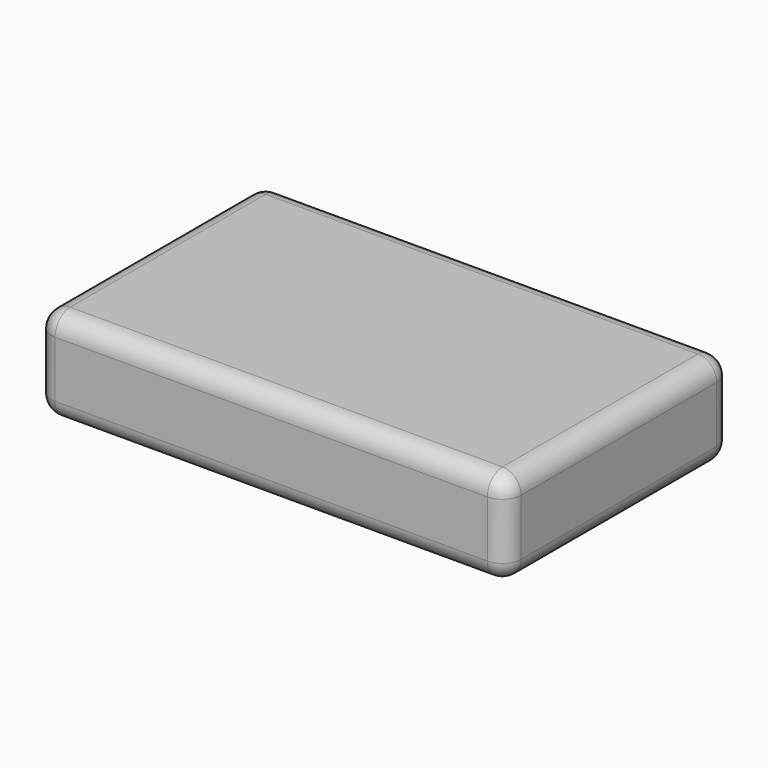
from build123d import *

# Parameters (mm, degrees)
F0_W         = 127
F0_H         = 76.2
F1_DEPTH     = 25.4
F2_R         = 5.08
F3_DEPTH     = 12.7
F4_W         = 101.6
F4_H         = 50.8
F5_DEPTH     = 12.7
F6_TEXT_SIZE = 70.5555555556
F7_DEPTH     = 22.86


# Not quite as in the source:
# - Text() gives the source's letters only with a copy of the font that has no kerning and outlines rounded to 1/6400 em; it was checked with that copy


with BuildPart() as f1:
    # F0 (on Top) → F1 (new body)
    with BuildSketch(Plane.XY):
        Rectangle(F0_W, F0_H)
    extrude(amount=F1_DEPTH)

    # F2
    f2_edges = [f1.edges().sort_by_distance(p)[0] for p in [
        (-63.5, 38.1, 12.7),
        (-63.5, 0, 25.4),
        (0, 38.1, 25.4),
        (0, -38.1, 25.4),
        (-63.5, -38.1, 12.7),
        (-63.5, 0, 0),
        (0, 38.1, 0),
        (63.5, 38.1, 12.7),
        (63.5, 0, 25.4),
        (63.5, 0, 0),
        (0, -38.1, 0),
        (63.5, -38.1, 12.7),
    ]]
    fillet(f2_edges, radius=F2_R)

    # F3 (cut): a face of the model
    f3_faces = [f1.faces().sort_by_distance(p)[0] for p in [
        (0, 0, 0),
    ]]
    extrude(f3_faces, amount=-F3_DEPTH, mode=Mode.SUBTRACT)

    # F4 (on face) → F5 (join)
    with BuildSketch(Plane(origin=(0, 0, 12.7), x_dir=(1, 0, 0), z_dir=(0, 0, -1))):
        Rectangle(F4_W, F4_H)
    extrude(amount=F5_DEPTH)

    # F6 (on face) → F7 (cut)
    with BuildSketch(Plane(origin=(0, 0, 0), x_dir=(1, 0, 0), z_dir=(0, 0, -1))):
        with Locations((-50.8, -25.4)):
            Text('AK', F6_TEXT_SIZE, font='Open Sans', font_style=FontStyle.BOLD, text_align=(TextAlign.LEFT, TextAlign.BOTTOM))
    extrude(amount=-F7_DEPTH, mode=Mode.SUBTRACT)


solid = f1.part
